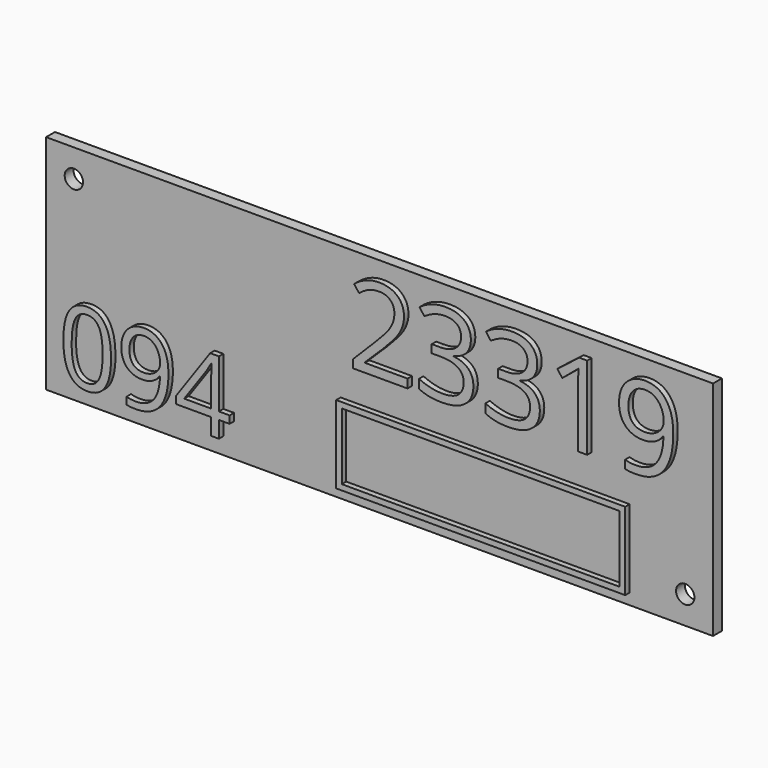
from build123d import *

# Parameters (mm, degrees)
F0_W         = 120
F0_H         = 40
F1_DEPTH     = 2
F3_D         = 3.3
F4_TEXT_SIZE = 20.9070615778
F5_DEPTH     = 1
F6_TEXT_SIZE = 18.1818181818
F7_DEPTH     = 1
F8_W         = 52
F8_H         = 14
F8_W_2       = 49.99999962
F8_H_2       = 11.99999962
F9_DEPTH     = 1


# Not quite as in the source:
# - Text() gives the source's letters only with a copy of the font that has no kerning and outlines rounded to 1/6400 em; it was checked with that copy


with BuildPart() as f1:
    # F0 (on Front) → F1 (new body)
    with BuildSketch(Plane.XZ):
        Rectangle(F0_W, F0_H)
    extrude(amount=F1_DEPTH)

    # F3 (through all)
    with Locations(Plane.XZ.offset(2)):
        with Locations((-55, 15), (55, -15)):
            Hole(F3_D / 2)

    # F4 (on face) → F5 (join)
    with BuildSketch(Plane.XZ.offset(2)):
        with Locations((-5, 2)):
            Text('23319', F4_TEXT_SIZE, font='Open Sans', text_align=(TextAlign.LEFT, TextAlign.BOTTOM))
    extrude(amount=F5_DEPTH)

    # F6 (on face) → F7 (join)
    with BuildSketch(Plane.XZ.offset(2)):
        with Locations((-57, -17)):
            Text('094', F6_TEXT_SIZE, font='Open Sans', text_align=(TextAlign.LEFT, TextAlign.BOTTOM))
    extrude(amount=F7_DEPTH)

    # F8 (on face) → F9 (join)
    with BuildSketch(Plane.XZ.offset(2)):
        with Locations((19, -11)):
            Rectangle(F8_W, F8_H)
        with Locations((19, -11)):
            Rectangle(F8_W_2, F8_H_2, mode=Mode.SUBTRACT)
    extrude(amount=F9_DEPTH)


solid = f1.part
